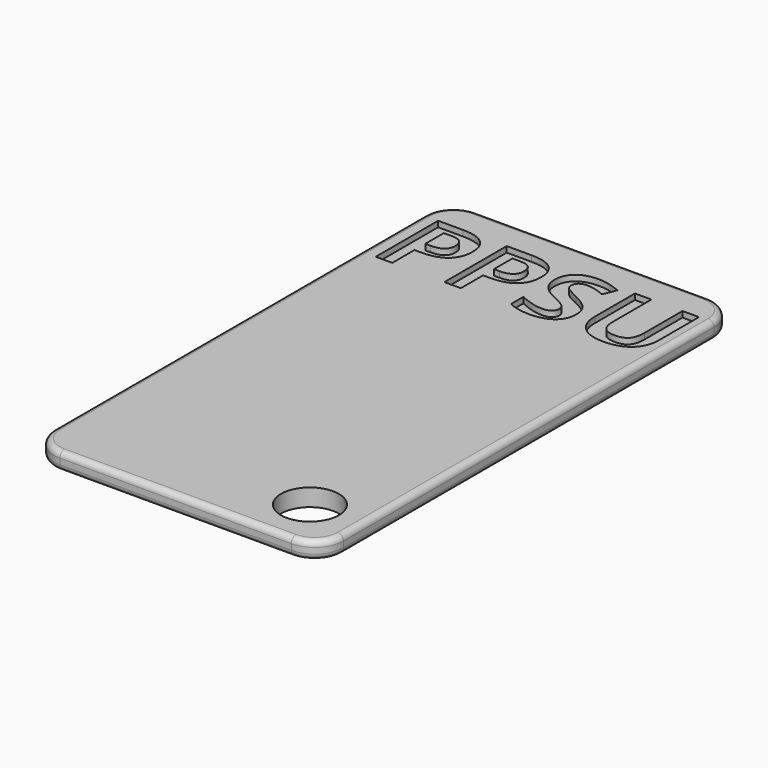
from build123d import *

# Parameters (mm, degrees)
F0_W         = 90
F0_H         = 50
F1_DEPTH     = 3
F2_R         = 1
F3_T1_DEPTH  = 3
F3_T4_ANGLE  = 90
F3_T6_ANGLE  = 90
F3_T8_ANGLE  = 90
F3_T10_ANGLE = 90
F3_T12_ANGLE = 90
F3_T14_ANGLE = 90
F3_T16_ANGLE = 90
F3_T18_ANGLE = 90
F5_ANGLE     = 90
F6_TEXT_SIZE = 18.8790560472
F7_DEPTH     = 1
F8_R         = 5
F9_DEPTH     = 3


# Not quite as in the source:
# - a fillet or chamfer that OpenCascade refuses, or shapes differently, is made with other operations: its cross-section is extruded or revolved along the edge and cut away or added
# - Text() gives the source's letters only with a copy of the font that has no kerning and outlines rounded to 1/6400 em; it was checked with that copy


with BuildPart() as f1:
    # F0 (on Top) → F1 (new body)
    with BuildSketch(Plane.XY):
        Rectangle(F0_W, F0_H)
    extrude(amount=F1_DEPTH)

    # F2
    f2_edges = [f1.edges().sort_by_distance(p)[0] for p in [
        (0, 25, 3),
        (-45, 0, 3),
        (0, -25, 3),
        (45, 0, 3),
        (0, 25, 0),
        (-45, 0, 0),
        (0, -25, 0),
        (45, 0, 0),
    ]]
    fillet(f2_edges, radius=F2_R)

    # F3: fillet of radius 5 on 4 edges, made by hand

    # F3_s2 → F3_t1 (cut)
    with BuildSketch(Plane.XY):
        with BuildLine():
            ThreePointArc((45, -20), (43.5355339059, -23.5355339059), (40, -25))
            Line((40, -25), (45, -25))
            Line((45, -25), (45, -20))
        make_face()
        with BuildLine():
            ThreePointArc((40, 25), (43.5355339059, 23.5355339059), (45, 20))
            Line((45, 20), (45, 25))
            Line((45, 25), (40, 25))
        make_face()
        with BuildLine():
            ThreePointArc((-40, 25), (-43.5355339059, 23.5355339059), (-45, 20))
            Line((-45, 20), (-45, 25))
            Line((-45, 25), (-40, 25))
        make_face()
        with BuildLine():
            ThreePointArc((-45, -20), (-43.5355339059, -23.5355339059), (-40, -25))
            Line((-40, -25), (-45, -25))
            Line((-45, -25), (-45, -20))
        make_face()
    extrude(amount=F3_T1_DEPTH, mode=Mode.SUBTRACT)

    # F3_s3 → F3_t4 (revolve, cut)
    with BuildSketch(Plane.YZ.offset(-40)):
        with BuildLine():
            ThreePointArc((-24, 0), (-24.7071067812, 0.2928932188), (-25, 1))
            Line((-25, 1), (-25, 0))
            Line((-25, 0), (-24, 0))
        make_face()
    revolve(axis=Axis((-40, -20, 0), (0, 0, -1)), revolution_arc=F3_T4_ANGLE, mode=Mode.SUBTRACT)

    # F3_s5 → F3_t6 (revolve, cut)
    with BuildSketch(Plane.XZ.offset(20)):
        with BuildLine():
            ThreePointArc((-44, 3), (-44.7071067812, 2.7071067812), (-45, 2))
            Line((-45, 2), (-45, 3))
            Line((-45, 3), (-44, 3))
        make_face()
    revolve(axis=Axis((-40, -20, 3), (0, 0, 1)), revolution_arc=F3_T6_ANGLE, mode=Mode.SUBTRACT)

    # F3_s7 → F3_t8 (revolve, cut)
    with BuildSketch(Plane.XZ.offset(-20)):
        with BuildLine():
            ThreePointArc((-44, 0), (-44.7071067812, 0.2928932188), (-45, 1))
            Line((-45, 1), (-45, 0))
            Line((-45, 0), (-44, 0))
        make_face()
    revolve(axis=Axis((-40, 20, 0), (0, 0, -1)), revolution_arc=F3_T8_ANGLE, mode=Mode.SUBTRACT)

    # F3_s9 → F3_t10 (revolve, cut)
    with BuildSketch(Plane.YZ.offset(-40)):
        with BuildLine():
            ThreePointArc((24, 3), (24.7071067812, 2.7071067812), (25, 2))
            Line((25, 2), (25, 3))
            Line((25, 3), (24, 3))
        make_face()
    revolve(axis=Axis((-40, 20, 3), (0, 0, 1)), revolution_arc=F3_T10_ANGLE, mode=Mode.SUBTRACT)

    # F3_s11 → F3_t12 (revolve, cut)
    with BuildSketch(Plane.YZ.offset(40)):
        with BuildLine():
            ThreePointArc((24, 0), (24.7071067812, 0.2928932188), (25, 1))
            Line((25, 1), (25, 0))
            Line((25, 0), (24, 0))
        make_face()
    revolve(axis=Axis((40, 20, 0), (0, 0, -1)), revolution_arc=F3_T12_ANGLE, mode=Mode.SUBTRACT)

    # F3_s13 → F3_t14 (revolve, cut)
    with BuildSketch(Plane.XZ.offset(-20)):
        with BuildLine():
            ThreePointArc((44, 3), (44.7071067812, 2.7071067812), (45, 2))
            Line((45, 2), (45, 3))
            Line((45, 3), (44, 3))
        make_face()
    revolve(axis=Axis((40, 20, 3), (0, 0, 1)), revolution_arc=F3_T14_ANGLE, mode=Mode.SUBTRACT)

    # F3_s15 → F3_t16 (revolve, cut)
    with BuildSketch(Plane.XZ.offset(20)):
        with BuildLine():
            ThreePointArc((44, 0), (44.7071067812, 0.2928932188), (45, 1))
            Line((45, 1), (45, 0))
            Line((45, 0), (44, 0))
        make_face()
    revolve(axis=Axis((40, -20, 0), (0, 0, -1)), revolution_arc=F3_T16_ANGLE, mode=Mode.SUBTRACT)

    # F3_s17 → F3_t18 (revolve, cut)
    with BuildSketch(Plane.YZ.offset(40)):
        with BuildLine():
            ThreePointArc((-24, 3), (-24.7071067812, 2.7071067812), (-25, 2))
            Line((-25, 2), (-25, 3))
            Line((-25, 3), (-24, 3))
        make_face()
    revolve(axis=Axis((40, -20, 3), (0, 0, 1)), revolution_arc=F3_T18_ANGLE, mode=Mode.SUBTRACT)


with BuildPart() as f1_1:
    # F5: moved
    add(f1.part.rotate(Axis((0, 0, 16.4477843791), (0, 0, 1)), F5_ANGLE))

    # F6 (on face) → F7 (cut)
    with BuildSketch(Plane.XY.offset(3)):
        with Locations((-24, 26.0923470388)):
            Text('PPSU', F6_TEXT_SIZE, font='Open Sans', font_style=FontStyle.BOLD, text_align=(TextAlign.LEFT, TextAlign.BOTTOM))
    extrude(amount=-F7_DEPTH, mode=Mode.SUBTRACT)

    # F8 (on face) → F9 (cut)
    with BuildSketch(Plane.XY.offset(3)):
        with Locations((16, -36)):
            Circle(F8_R)
    extrude(amount=-F9_DEPTH, mode=Mode.SUBTRACT)


solid = f1_1.part
